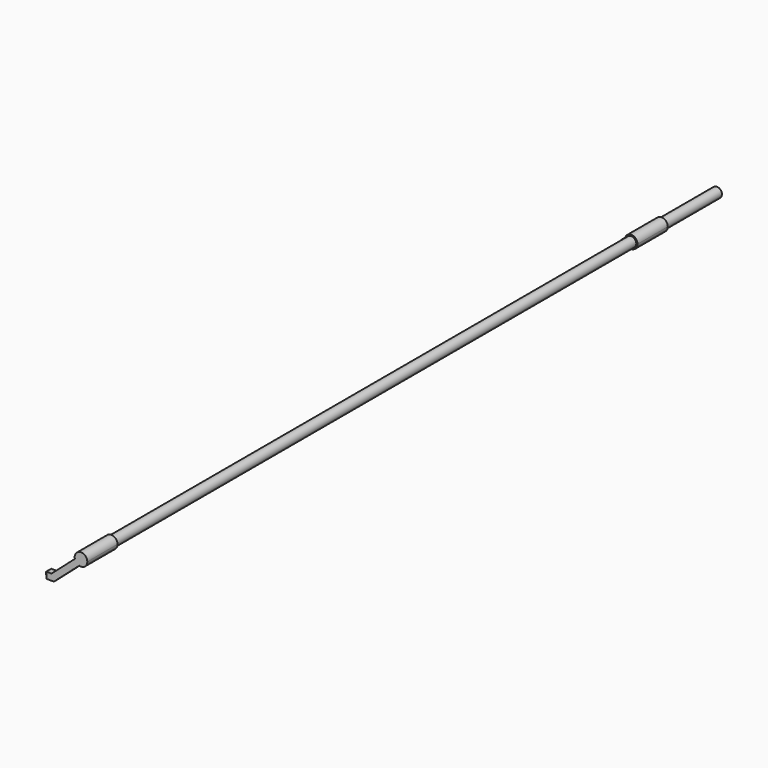
from build123d import *

# Parameters (mm, degrees)
F2_DEPTH  = 30
F3_DEPTH  = 5
F5_DEPTH  = 30
F6_DEPTH  = 5
F7_T      = -1
F8_T      = -1
F9_R      = 4
F10_DEPTH = 630
F6_FACE_W = 5
F6_FACE_H = 5
F3_FACE_W = 5
F3_FACE_H = 5
F14_R     = 1.5
F15_DEPTH = 3
F16_R     = 1.5
F17_DEPTH = 3
F18_DEPTH = 4
F19_DEPTH = 4


with BuildPart() as f2:
    # F1 (on Front) → F2 (new body)
    with BuildSketch(Plane.XZ):
        with BuildLine():
            ThreePointArc((-1.3935307675, -4.801882131), (3.0026943037, -3.9979778537), (5, 0))
            ThreePointArc((5, 0), (-0.6014206199, 4.9636975369), (-4.8553172952, -1.1941080199))
            ThreePointArc((-4.8553172952, -1.1941080199), (-3.6077741111, -3.4617865277), (-1.3935307675, -4.801882131))
        make_face()
    extrude(amount=F2_DEPTH)

    # F1 (on Front) → F3 (join)
    with BuildSketch(Plane.XZ):
        with BuildLine():
            ThreePointArc((-1.3935307675, -4.801882131), (-3.6077741111, -3.4617865277), (-4.8553172952, -1.1941080199))
            Line((-4.8553172952, -1.1941080199), (-12.3652843317, -7.7971675463))
            Line((-12.3652843317, -7.7971675463), (-8.903497804, -11.4049416575))
            Line((-8.903497804, -11.4049416575), (-1.3935307675, -4.801882131))
        make_face()
    extrude(amount=F3_DEPTH)

    # F8
    f8_openings = [f2.faces().sort_by_distance(p)[0] for p in [
        (0, -30, 0),
    ]]
    offset(amount=F8_T, openings=f8_openings)

    # F13: sweep along a path in F11
    with BuildLine(Plane.XZ.offset(576)) as f13_path:
        Line((0, 0), (-22.5299011097, -19.8091785794))
        Line((-22.5299011097, -19.8091785794), (-27.5299011097, -19.8091785794))
    # F3_face (on face) → F13 (sweep)
    with BuildSketch(Plane(origin=(-10.6343910679, -2.5, -9.6010546019), x_dir=(0, -1, 0), z_dir=(-0.7215548222, 0, -0.6923573055))):
        Rectangle(F3_FACE_W, F3_FACE_H)
    sweep(path=f13_path.line, transition=Transition.RIGHT)

    # F16 (on face) → F17 (cut)
    with BuildSketch(Plane(origin=(-28.3388841018, 0, -1.234225183), x_dir=(0, -1, 0), z_dir=(-0.9990529432, 0, -0.0435111099))):
        with Locations((2.5, -18.7811488439)):
            Circle(F16_R)
    extrude(amount=-F17_DEPTH, mode=Mode.SUBTRACT)

    # F18 (add): a face of the model
    f18_faces = [f2.faces().sort_by_distance(p)[0] for p in [
        (-24.5245366401, -2.5, -19.8670538823),
    ]]
    extrude(f18_faces, amount=F18_DEPTH)


with BuildPart() as f5:
    # F4 (on offset) → F5 (new body)
    with BuildSketch(Plane.XZ.offset(576)):
        with BuildLine():
            ThreePointArc((-1.3935307675, -4.801882131), (3.0026943037, -3.9979778537), (5, 0))
            ThreePointArc((5, 0), (-0.6014206199, 4.9636975369), (-4.8553172952, -1.1941080199))
            ThreePointArc((-4.8553172952, -1.1941080199), (-3.6077741111, -3.4617865277), (-1.3935307675, -4.801882131))
        make_face()
    extrude(amount=-F5_DEPTH)

    # F4 (on offset) → F6 (join)
    with BuildSketch(Plane.XZ.offset(576)):
        with BuildLine():
            ThreePointArc((-1.3935307675, -4.801882131), (-3.6077741111, -3.4617865277), (-4.8553172952, -1.1941080199))
            Line((-4.8553172952, -1.1941080199), (-12.3652843317, -7.7971675463))
            Line((-12.3652843317, -7.7971675463), (-8.903497804, -11.4049416575))
            Line((-8.903497804, -11.4049416575), (-1.3935307675, -4.801882131))
        make_face()
    extrude(amount=-F6_DEPTH)

    # F7
    f7_openings = [f5.faces().sort_by_distance(p)[0] for p in [
        (0, -546, 0),
    ]]
    offset(amount=F7_T, openings=f7_openings)

    # F12: sweep along a path in F11
    with BuildLine(Plane.XZ.offset(576)) as f12_path:
        Line((0, 0), (-22.5299011097, -19.8091785794))
        Line((-22.5299011097, -19.8091785794), (-27.5299011097, -19.8091785794))
    # F6_face (on face) → F12 (sweep)
    with BuildSketch(Plane(origin=(-10.6343910679, -573.5, -9.6010546019), x_dir=(0, -1, 0), z_dir=(-0.7215548222, 0, -0.6923573055))):
        Rectangle(F6_FACE_W, F6_FACE_H)
    sweep(path=f12_path.line, transition=Transition.RIGHT)

    # F14 (on face) → F15 (cut)
    with BuildSketch(Plane(origin=(-28.3388841018, 0, -1.234225183), x_dir=(0, -1, 0), z_dir=(-0.9990529432, 0, -0.0435111099))):
        with Locations((573.5, -18.7811488439)):
            Circle(F14_R)
    extrude(amount=-F15_DEPTH, mode=Mode.SUBTRACT)

    # F19 (add): a face of the model
    f19_faces = [f5.faces().sort_by_distance(p)[0] for p in [
        (-24.5245366401, -573.5, -19.8670538823),
    ]]
    extrude(f19_faces, amount=F19_DEPTH)


with BuildPart() as f10:
    # F9 (on face) → F10 (new body)
    with BuildSketch(Plane(origin=(0, -575, 0), x_dir=(-1, 0, 0), z_dir=(0, 1, 0))):
        Circle(F9_R)
    extrude(amount=F10_DEPTH)


solid = Compound([f2.part, f5.part, f10.part])
